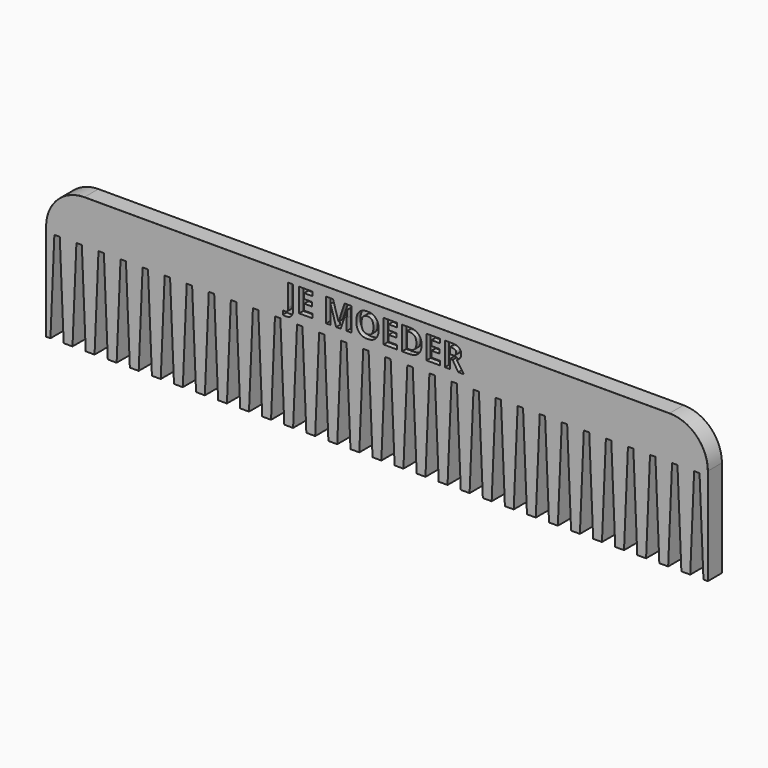
from build123d import *

# Parameters (mm, degrees)
F1_DEPTH     = 2
F2_R         = 8.6911688245
F4_R         = 0.0241421356
F5_TEXT_SIZE = 7.4786315155
F6_DEPTH     = 1.2


# Not quite as in the source:
# - Text() gives the source's letters only with a copy of the font that has no kerning and outlines rounded to 1/6400 em; it was checked with that copy


with BuildPart() as f1:
    # F0 (on Front) → F1 (new body, symmetric)
    with BuildSketch(Plane.XZ):
        Polygon((0, 30.6657277333), (0, 0), (1, 0), (1.8870279845, 20.949518308), (3.1129720155, 20.949518308), (4, 0), (6, 0), (6.8870279845, 20.949518308), (8.1129720155, 20.949518308), (9, 0), (11, 0), (11.8870279845, 20.949518308), (13.1129720155, 20.949518308), (14, 0), (16, 0), (16.8870279845, 20.949518308), (18.1129720155, 20.949518308), (19, 0), (21, 0), (21.8870279845, 20.949518308), (23.1129720155, 20.949518308), (24, 0), (26, 0), (26.8870279845, 20.949518308), (28.1129720155, 20.949518308), (29, 0), (31, 0), (31.8870279845, 20.949518308), (33.1129720155, 20.949518308), (34, 0), (36, 0), (36.8870279845, 20.949518308), (38.1129720155, 20.949518308), (39, 0), (41, 0), (41.8870279845, 20.949518308), (43.1129720155, 20.949518308), (44, 0), (46, 0), (46.8870279845, 20.949518308), (48.1129720155, 20.949518308), (49, 0), (51, 0), (51.8870279845, 20.949518308), (53.1129720155, 20.949518308), (54, 0), (56, 0), (56.8870279845, 20.949518308), (58.1129720155, 20.949518308), (59, 0), (61, 0), (61.8870279845, 20.949518308), (63.1129720155, 20.949518308), (64, 0), (66, 0), (66.8870279845, 20.949518308), (68.1129720155, 20.949518308), (69, 0), (71, 0), (71.8870279845, 20.949518308), (73.1129720155, 20.949518308), (74, 0), (75, 0), (75, 30.6657277333), align=None)
    extrude(amount=F1_DEPTH, both=True)

    # F2
    f2_edges = [f1.edges().sort_by_distance(p)[0] for p in [
        (75, 0, 30.665728),
    ]]
    fillet(f2_edges, radius=F2_R)

    # F3: F1 across plane


with BuildPart() as f1_1:
    add(f1.part)
    add(f1.part.mirror(Plane.YZ))

    # F4
    f4_edges = [f1_1.edges().sort_by_distance(p)[0] for p in [
        (0, -2, 30.665728),
        (0, 2, 30.665728),
        (72.454416, -2, 28.120143),
        (75, -2, 10.987279),
        (-75, -2, 10.987279),
        (-72.454416, -2, 28.120143),
        (-72.454416, 2, 28.120143),
        (-75, 2, 10.987279),
        (72.454416, 2, 28.120143),
        (75, 2, 10.987279),
    ]]
    fillet(f4_edges, radius=F4_R)

    # F5 (on face) → F6 (cut)
    with BuildSketch(Plane.XZ.offset(2)):
        with Locations((-20.7812506706, 23.3052931726)):
            Text('JE MOEDER', F5_TEXT_SIZE, font='Open Sans', font_style=FontStyle.BOLD, text_align=(TextAlign.LEFT, TextAlign.BOTTOM))
    extrude(amount=-F6_DEPTH, mode=Mode.SUBTRACT)


solid = f1_1.part
